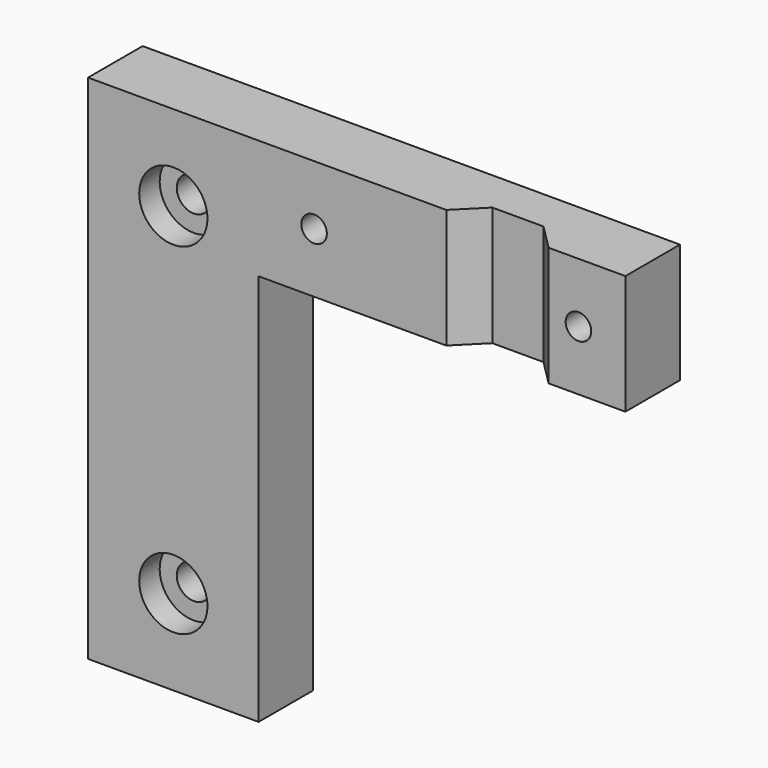
from build123d import *

# Parameters (mm, degrees)
F1_DEPTH = 14
F0_W     = 20
F0_H     = 8
F2_DEPTH = 60
F3_R     = 4
F3_R_2   = 2
F3_R_3   = 1.5
F4_DEPTH = 8.001
F5_DEPTH = 3
F6_DEPTH = 5


# Not quite as in the source:
# - a feature names something its author has since deleted; it is built from what else it names


with BuildPart() as f1:
    # F0 (on Top) → F1 (new body)
    with BuildSketch(Plane.XY):
        Polygon((43, 0), (43, 8), (0, 8), (0, 0), (22, 0), (25, 3), (31, 3), (34, 0), align=None)
    extrude(amount=-F1_DEPTH)

    # F0 (on Top) → F2 (join)
    with BuildSketch(Plane.XY):
        with Locations((-10, 4)):
            Rectangle(F0_W, F0_H)
    extrude(amount=-F2_DEPTH)

    # F3 (on face) → F4 (cut, through all)
    with BuildSketch(Plane(origin=(0, 8, 0), x_dir=(-1, 0, 0), z_dir=(0, 1, 0))):
        with Locations((10, -10)):
            Circle(F3_R)
        with Locations((10, -10)):
            Circle(F3_R_2, mode=Mode.SUBTRACT)
        with Locations((10, -50)):
            Circle(F3_R)
        with Locations((10, -50)):
            Circle(F3_R_2, mode=Mode.SUBTRACT)
        with Locations((10, -10)):
            Circle(F3_R_2)
        with Locations((10, -50)):
            Circle(F3_R_2)
        with Locations((-37.5, -7)):
            Circle(F3_R_3)
        with Locations((-6.5, -7)):
            Circle(F3_R_3)
    extrude(amount=-F4_DEPTH, mode=Mode.SUBTRACT)

    # F3 (on face) → F5 (cut)
    with BuildSketch(Plane(origin=(0, 8, 0), x_dir=(-1, 0, 0), z_dir=(0, 1, 0))):
        Polygon((-8.1743157806, -9.9), (-4.8256842194, -9.9), (-3.1513684387, -7), (-4.8256842194, -4.1), (-8.1743157806, -4.1), (-9.8486315613, -7), align=None)
        with Locations((-6.5, -7)):
            Circle(F3_R_3, mode=Mode.SUBTRACT)
        Polygon((-39.1743157806, -9.9), (-35.8256842194, -9.9), (-34.1513684387, -7), (-35.8256842194, -4.1), (-39.1743157806, -4.1), (-40.8486315613, -7), align=None)
        with Locations((-37.5, -7)):
            Circle(F3_R_3, mode=Mode.SUBTRACT)
    extrude(amount=-F5_DEPTH, mode=Mode.SUBTRACT)

    # F3 (on face) → F6 (join)
    with BuildSketch(Plane(origin=(0, 8, 0), x_dir=(-1, 0, 0), z_dir=(0, 1, 0))):
        with Locations((10, -10)):
            Circle(F3_R)
        with Locations((10, -10)):
            Circle(F3_R_2, mode=Mode.SUBTRACT)
        with Locations((10, -50)):
            Circle(F3_R)
        with Locations((10, -50)):
            Circle(F3_R_2, mode=Mode.SUBTRACT)
    extrude(amount=-F6_DEPTH)


solid = f1.part
